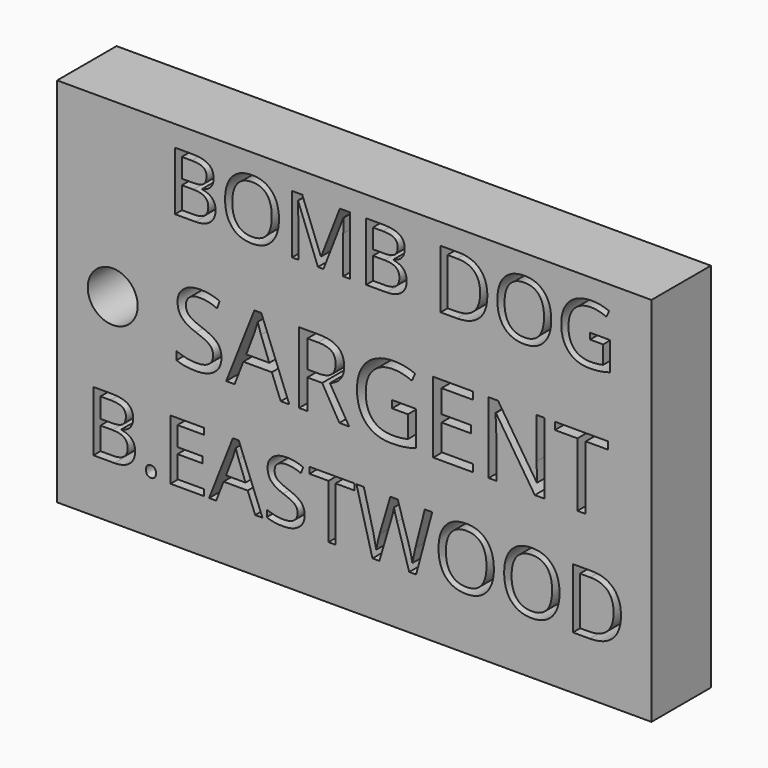
from build123d import *

# Parameters (mm, degrees)
F0_W           = 40
F0_H           = 25
F0_R           = 1.6818068079
F1_DEPTH       = 5
F2_TEXT_SIZE   = 6.7081541703
F2_TEXT_SIZE_2 = 5.6728746535
F2_TEXT_SIZE_3 = 5.5214412795
F3_DEPTH       = 3


# Not quite as in the source:
# - Text() gives the source's letters only with a copy of the font that has no kerning and outlines rounded to 1/6400 em; it was checked with that copy


with BuildPart() as f1:
    # F0 (on Front) → F1 (new body)
    with BuildSketch(Plane.XZ):
        with Locations((-9.2133465409, -3.5545930266)):
            Rectangle(F0_W, F0_H)
        with Locations((-25.4701972008, -2.6517000515)):
            Circle(F0_R, mode=Mode.SUBTRACT)
    extrude(amount=F1_DEPTH)

    # F2 (on face) → F3 (cut)
    with BuildSketch(Plane.XZ.offset(5)):
        with Locations((-21.515045315, -5.1693867426)):
            Text('SARGENT', F2_TEXT_SIZE, font='Open Sans', text_align=(TextAlign.LEFT, TextAlign.BOTTOM))
        with Locations((-27.325136587, -12.4719934538)):
            Text('B.EASTWOOD', F2_TEXT_SIZE_2, font='Open Sans', text_align=(TextAlign.LEFT, TextAlign.BOTTOM))
        with Locations((-21.8230551109, 3.5977147054)):
            Text('BOMB DOG', F2_TEXT_SIZE_3, font='Open Sans', text_align=(TextAlign.LEFT, TextAlign.BOTTOM))
    extrude(amount=-F3_DEPTH, mode=Mode.SUBTRACT)


solid = f1.part
